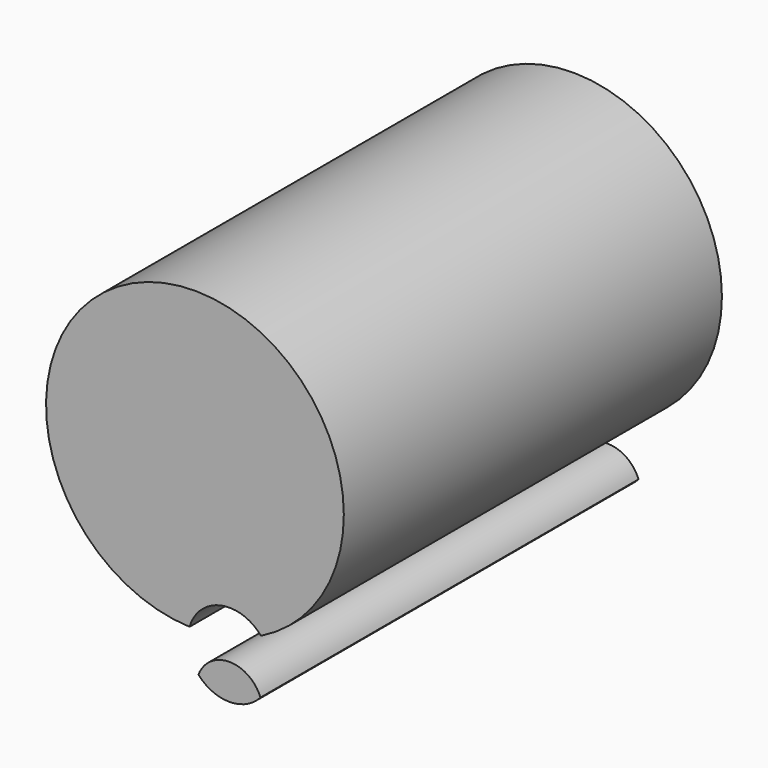
from build123d import *

# Parameters (mm, degrees)
F1_DEPTH = 203.2


# Not quite as in the source:
# - a feature names something its author has since deleted; it is built from what else it names


with BuildPart() as f1:
    # F0 (on Front) → F1 (new body)
    with BuildSketch(Plane.XZ):
        with BuildLine():
            ThreePointArc((-67.802701422, -17.997257176), (-54.417922901, -5.5408285068), (-37.0972669354, -11.3982842828))
            ThreePointArc((-37.0972669354, -11.3982842828), (-78.9414112036, 108.5684996634), (-67.802701422, -17.997257176))
        make_face()
    extrude(amount=F1_DEPTH)


with BuildPart() as f1b:
    # F0 (on Front) → F1, piece 2 (new body)
    with BuildSketch(Plane.XZ):
        with BuildLine():
            ThreePointArc((-37.333307052, -34.8517759394), (-50.6679601967, -25.6607035221), (-64.0026133414, -34.8517759394))
            ThreePointArc((-64.0026133414, -34.8517759394), (-50.6679601967, -40.8368594944), (-37.333307052, -34.8517759394))
        make_face()
    extrude(amount=F1_DEPTH)


solid = Compound([f1.part, f1b.part])
